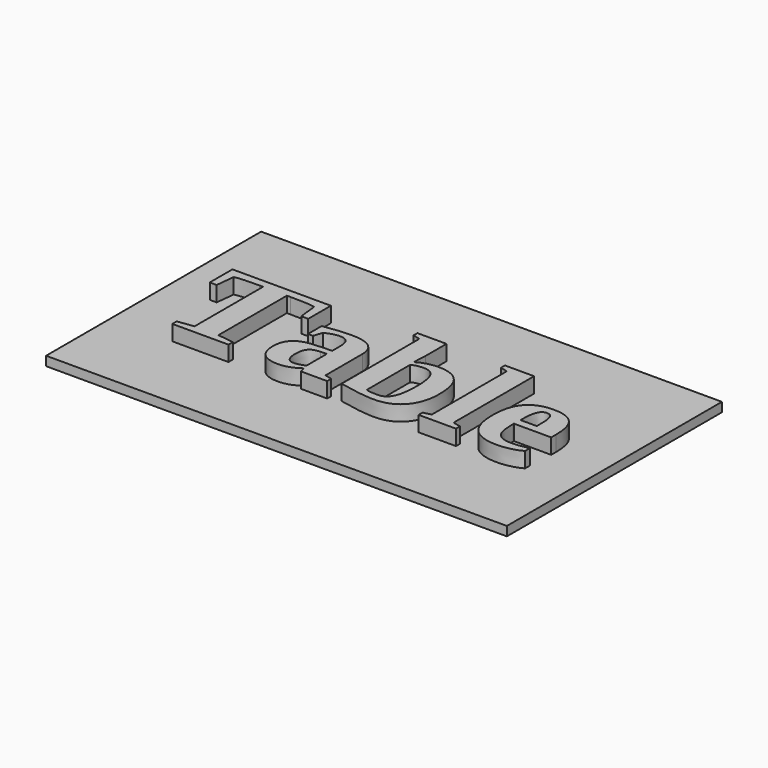
from build123d import *

# Parameters (mm, degrees)
F0_W         = 60
F0_H         = 35
F1_DEPTH     = 1.2
F2_TEXT_SIZE = 20.1498646181
F3_DEPTH     = 2


# Not quite as in the source:
# - Text() gives the source's letters only with a copy of the font that has no kerning and outlines rounded to 1/6400 em; it was checked with that copy


with BuildPart() as f1:
    # F0 (on Top) → F1 (new body)
    with BuildSketch(Plane.XY):
        with Locations((30, 17.5)):
            Rectangle(F0_W, F0_H)
    extrude(amount=F1_DEPTH)

    # F2 (on face) → F3 (join)
    with BuildSketch(Plane.XY.offset(1.2)):
        with Locations((5, 10.492097475)):
            Text('Table', F2_TEXT_SIZE, font='Tinos', font_style=FontStyle.BOLD, text_align=(TextAlign.LEFT, TextAlign.BOTTOM))
    extrude(amount=F3_DEPTH)


solid = f1.part
